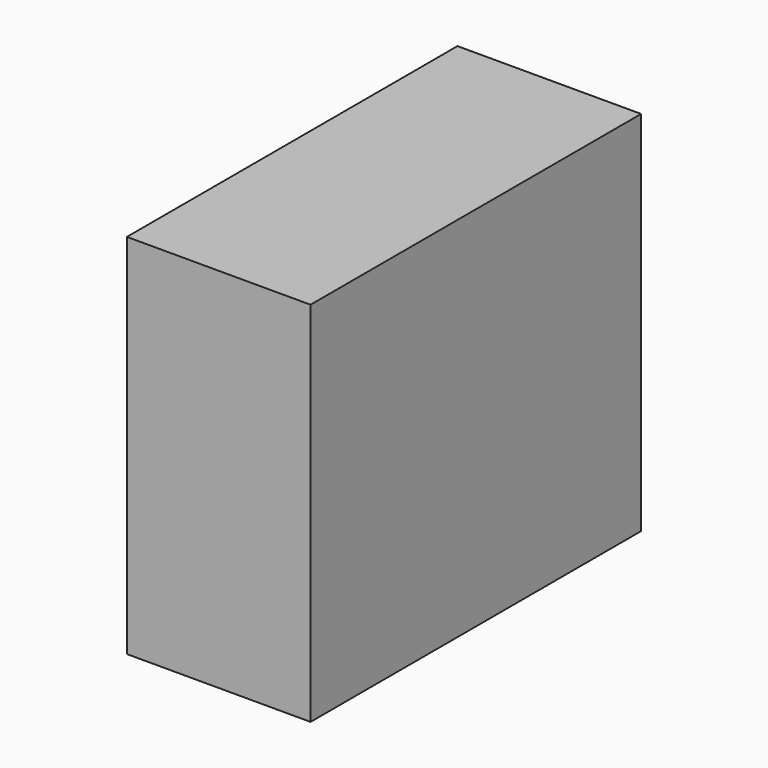
from build123d import *

# Parameters (mm, degrees)
F0_W     = 2
F0_H     = 4.5
F1_DEPTH = 4


# Not quite as in the source:
# - a feature names something its author has since deleted; it is built from what else it names


with BuildPart() as f1:
    # F0 (on Top) → F1 (new body)
    with BuildSketch(Plane.XY):
        with Locations((0.0788692376, -16.949905917)):
            Rectangle(F0_W, F0_H)
    extrude(amount=F1_DEPTH)


solid = f1.part
